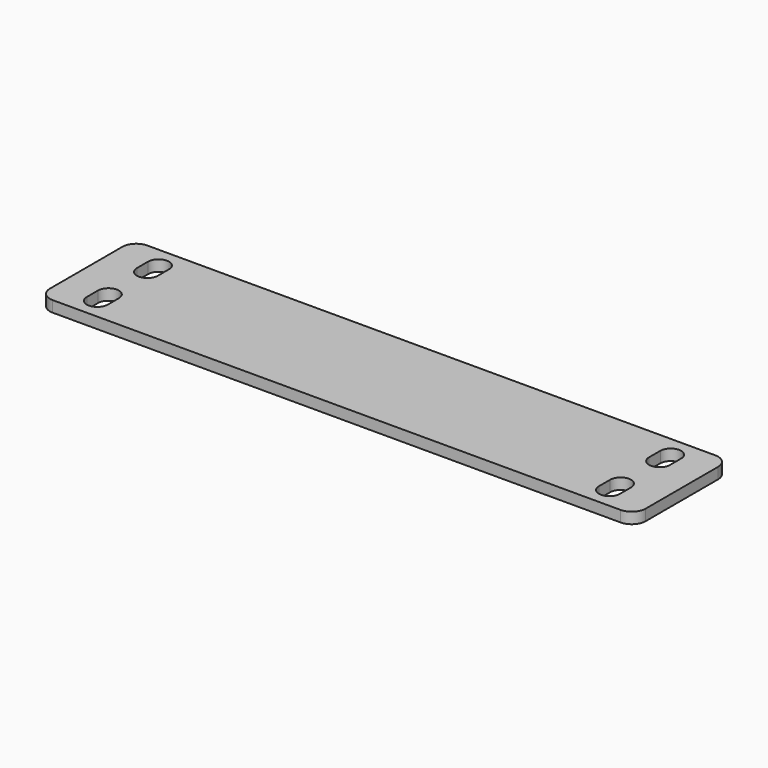
from build123d import *

# Parameters (mm, degrees)
F0_W     = 85.6
F0_H     = 17
F1_DEPTH = 1.5875
F2_R     = 2


# Not quite as in the source:
# - a length typed as a fraction of an inch, garbled in the dataset ("3 / 203.2 mm" for 3/8 in), is restored


with BuildPart() as f1:
    # F0 (on Top) → F1 (new body)
    with BuildSketch(Plane.XY):
        Rectangle(F0_W, F0_H)
        with BuildLine():
            ThreePointArc((-35.3, -5.5), (-36.8, -7), (-38.3, -5.5))
            Line((-38.3, -5.5), (-38.3, -3.5))
            ThreePointArc((-38.3, -3.5), (-36.8, -2), (-35.3, -3.5))
            Line((-35.3, -3.5), (-35.3, -5.5))
        make_face(mode=Mode.SUBTRACT)
        with BuildLine():
            ThreePointArc((35.3, -3.5), (36.8, -2), (38.3, -3.5))
            Line((38.3, -3.5), (38.3, -5.5))
            ThreePointArc((38.3, -5.5), (36.8, -7), (35.3, -5.5))
            Line((35.3, -5.5), (35.3, -3.5))
        make_face(mode=Mode.SUBTRACT)
        with BuildLine():
            ThreePointArc((-38.3, 5.5), (-36.8, 7), (-35.3, 5.5))
            Line((-35.3, 5.5), (-35.3, 3.5))
            ThreePointArc((-35.3, 3.5), (-36.8, 2), (-38.3, 3.5))
            Line((-38.3, 3.5), (-38.3, 5.5))
        make_face(mode=Mode.SUBTRACT)
        with BuildLine():
            Line((35.3, 3.5), (35.3, 5.5))
            ThreePointArc((35.3, 5.5), (36.8, 7), (38.3, 5.5))
            Line((38.3, 5.5), (38.3, 3.5))
            ThreePointArc((38.3, 3.5), (36.8, 2), (35.3, 3.5))
        make_face(mode=Mode.SUBTRACT)
    extrude(amount=F1_DEPTH)

    # F2
    f2_edges = [f1.edges().sort_by_distance(p)[0] for p in [
        (-42.8, -8.5, 0.79375),
        (-42.8, 8.5, 0.79375),
        (42.8, 8.5, 0.79375),
        (42.8, -8.5, 0.79375),
    ]]
    fillet(f2_edges, radius=F2_R)


solid = f1.part
